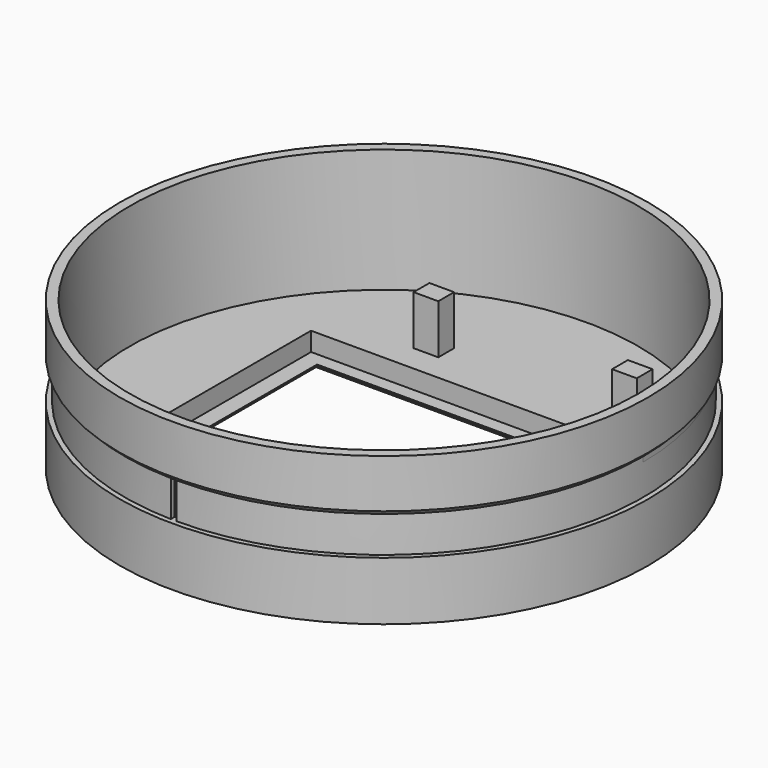
from build123d import *

# Parameters (mm, degrees)
F0_R        = 67.945
F1_DEPTH    = 38.1
F2_R        = 65.405
F3_DEPTH    = 31.75
F5_W        = 2.54
F5_H        = 8.001
F7_S5_R     = 66.675
F7_T6_DEPTH = 98
F8_W        = 73.66
F8_H        = 49.022
F9_DEPTH    = 6.351
F10_W       = 85.852
F10_H       = 56.007
F11_DEPTH   = 4.826
F12_W       = 5.08
F12_H       = 53.34
F13_DEPTH   = 4.826
F14_SIZE    = 1.27
F15_W       = 1.524
F15_H       = 9.271
F16_DEPTH   = 67.946
F17_W       = 6.35
F17_H       = 5.08
F18_DEPTH   = 12.7


# Not quite as in the source:
# - a fillet or chamfer that OpenCascade refuses, or shapes differently, is made with other operations: its cross-section is extruded or revolved along the edge and cut away or added


with BuildPart() as f1:
    # F0 (on Top) → F1 (new body)
    with BuildSketch(Plane.XY):
        Circle(F0_R)
    extrude(amount=-F1_DEPTH)

    # F2 (on face) → F3 (cut)
    with BuildSketch(Plane.XY):
        Circle(F2_R)
    extrude(amount=-F3_DEPTH, mode=Mode.SUBTRACT)

    # F5 (on Front) → F6 (revolve, cut)
    with BuildSketch(Plane.XZ):
        with Locations((-67.945, -19.05)):
            Rectangle(F5_W, F5_H)
    revolve(axis=Axis((0, 0, 0), (0, 0, 1)), mode=Mode.SUBTRACT)

    # F7: chamfer of 2.54 on 1 edges, made by hand


with BuildPart() as f7_tool2:
    # F7_s3 → F7_t4 (revolve)
    with BuildSketch(Plane.XZ):
        Polygon((67.945, -12.5095), (65.405, -15.0495), (67.945, -15.0495), align=None)
    revolve(axis=Axis((0, 0, -15.0495), (0, 0, 1)))

    # F7_s5 → F7_t6 (cut, symmetric)
    with BuildSketch(Plane.XY.offset(-13.8)):
        Circle(F7_S5_R)
    extrude(amount=F7_T6_DEPTH, both=True, mode=Mode.SUBTRACT)


with BuildPart() as f1_1:
    add(f1.part)

    # F7_t1: cut F7_tool2
    add(f7_tool2.part, mode=Mode.SUBTRACT)

    # F8 (on face) → F9 (cut, through all)
    with BuildSketch(Plane.XY.offset(-31.75)):
        Rectangle(F8_W, F8_H)
    extrude(amount=-F9_DEPTH, mode=Mode.SUBTRACT)

    # F10 (on face) → F11 (cut, through all)
    with BuildSketch(Plane.XY.offset(-31.75)):
        with Locations((1.75, 0)):
            Rectangle(F10_W, F10_H)
    extrude(amount=-F11_DEPTH, mode=Mode.SUBTRACT)

    # F12 (on face) → F13 (cut, through all)
    with BuildSketch(Plane.XY.offset(-31.75)):
        with Locations((47.216, 0)):
            Rectangle(F12_W, F12_H)
    extrude(amount=-F13_DEPTH, mode=Mode.SUBTRACT)

    # F14
    f14_edges = [f1_1.edges().sort_by_distance(p)[0] for p in [
        (0, 24.511, -38.1),
        (-36.83, 0, -38.1),
        (36.83, 0, -38.1),
        (0, -24.511, -38.1),
    ]]
    chamfer(f14_edges, length=F14_SIZE)

    # F15 (on Front) → F16 (cut, through all)
    with BuildSketch(Plane.XZ):
        with Locations((-0.762, -18.415)):
            Rectangle(F15_W, F15_H)
    extrude(amount=F16_DEPTH, mode=Mode.SUBTRACT)

    # F17 (on face) → F18 (join)
    with BuildSketch(Plane.XY.offset(-31.75)):
        with Locations((-17.145, 37.465)):
            Rectangle(F17_W, F17_H)
        with Locations((34.925, 36.195)):
            Rectangle(F17_W, F17_H)
        with Locations((-15.875, -43.505)):
            Rectangle(F17_W, F17_H)
        with Locations((34.925, -38.735)):
            Rectangle(F17_W, F17_H)
    extrude(amount=F18_DEPTH)


solid = f1_1.part
